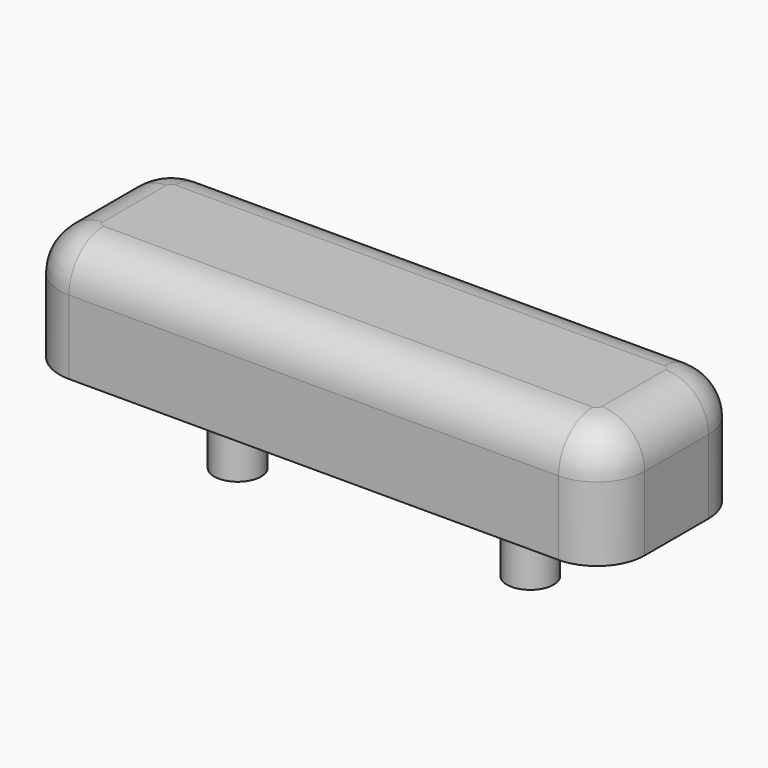
from build123d import *

# Parameters (mm, degrees)
F0_W         = 50
F0_H         = 15
F0_R         = 2
F1_DEPTH     = 10
F2_R         = 3.6792614691
F3_T1_DEPTH  = 20.2290713461
F3_T4_ANGLE  = 90
F3_T6_ANGLE  = 90
F3_T8_ANGLE  = 90
F3_T10_ANGLE = 90
F4_D         = 4.5
F4_DEPTH     = 0.5
F4_TIP       = 1.3519363928
F5_DEPTH     = 7


# Not quite as in the source:
# - a fillet or chamfer that OpenCascade refuses, or shapes differently, is made with other operations: its cross-section is extruded or revolved along the edge and cut away or added


with BuildPart() as f1:
    # F0 (on Top) → F1 (new body)
    with BuildSketch(Plane.XY):
        Rectangle(F0_W, F0_H)
        with Locations((-12.5, 0)):
            Circle(F0_R, mode=Mode.SUBTRACT)
        with Locations((12.5, 0)):
            Circle(F0_R, mode=Mode.SUBTRACT)
        with Locations((12.5, 0)):
            Circle(F0_R)
        with Locations((-12.5, 0)):
            Circle(F0_R)
    extrude(amount=F1_DEPTH)

    # F2
    f2_edges = [f1.edges().sort_by_distance(p)[0] for p in [
        (0, -7.5, 10),
        (-25, 0, 10),
        (25, 0, 10),
        (0, 7.5, 10),
    ]]
    fillet(f2_edges, radius=F2_R)

    # F3: fillet of radius 4.0916285384 on 4 edges, made by hand

    # F3_s2 → F3_t1 (cut)
    with BuildSketch(Plane.XY.offset(-10.2290713461)):
        with BuildLine():
            ThreePointArc((-20.9083714616, 7.5), (-23.8015897472, 6.3015897472), (-25, 3.4083714616))
            Line((-25, 3.4083714616), (-25, 7.5))
            Line((-25, 7.5), (-20.9083714616, 7.5))
        make_face()
        with BuildLine():
            ThreePointArc((-20.9083714616, -7.5), (-23.8015897472, -6.3015897472), (-25, -3.4083714616))
            Line((-25, -3.4083714616), (-25, -7.5))
            Line((-25, -7.5), (-20.9083714616, -7.5))
        make_face()
        with BuildLine():
            ThreePointArc((25, 3.4083714616), (23.8015897472, 6.3015897472), (20.9083714616, 7.5))
            Line((20.9083714616, 7.5), (25, 7.5))
            Line((25, 7.5), (25, 3.4083714616))
        make_face()
        with BuildLine():
            ThreePointArc((25, -3.4083714616), (23.8015897472, -6.3015897472), (20.9083714616, -7.5))
            Line((20.9083714616, -7.5), (25, -7.5))
            Line((25, -7.5), (25, -3.4083714616))
        make_face()
    extrude(amount=F3_T1_DEPTH, mode=Mode.SUBTRACT)

    # F3_s3 → F3_t4 (revolve, cut)
    with BuildSketch(Plane.YZ.offset(20.9083714616)):
        with BuildLine():
            ThreePointArc((-3.8207385309, 10), (-6.4223692655, 8.9223692655), (-7.5, 6.3207385309))
            Line((-7.5, 6.3207385309), (-7.5, 10))
            Line((-7.5, 10), (-3.8207385309, 10))
        make_face()
    revolve(axis=Axis((20.9083714616, -3.4083714616, 10), (0, 0, 1)), revolution_arc=F3_T4_ANGLE, mode=Mode.SUBTRACT)

    # F3_s5 → F3_t6 (revolve, cut)
    with BuildSketch(Plane.XZ.offset(-3.4083714616)):
        with BuildLine():
            ThreePointArc((21.3207385309, 10), (23.9223692655, 8.9223692655), (25, 6.3207385309))
            Line((25, 6.3207385309), (25, 10))
            Line((25, 10), (21.3207385309, 10))
        make_face()
    revolve(axis=Axis((20.9083714616, 3.4083714616, 10), (0, 0, 1)), revolution_arc=F3_T6_ANGLE, mode=Mode.SUBTRACT)

    # F3_s7 → F3_t8 (revolve, cut)
    with BuildSketch(Plane.XZ.offset(3.4083714616)):
        with BuildLine():
            ThreePointArc((-21.3207385309, 10), (-23.9223692655, 8.9223692655), (-25, 6.3207385309))
            Line((-25, 6.3207385309), (-25, 10))
            Line((-25, 10), (-21.3207385309, 10))
        make_face()
    revolve(axis=Axis((-20.9083714616, -3.4083714616, 10), (0, 0, 1)), revolution_arc=F3_T8_ANGLE, mode=Mode.SUBTRACT)

    # F3_s9 → F3_t10 (revolve, cut)
    with BuildSketch(Plane.YZ.offset(-20.9083714616)):
        with BuildLine():
            ThreePointArc((3.8207385309, 10), (6.4223692655, 8.9223692655), (7.5, 6.3207385309))
            Line((7.5, 6.3207385309), (7.5, 10))
            Line((7.5, 10), (3.8207385309, 10))
        make_face()
    revolve(axis=Axis((-20.9083714616, 3.4083714616, 10), (0, 0, 1)), revolution_arc=F3_T10_ANGLE, mode=Mode.SUBTRACT)

    # F4
    with Locations(Plane(origin=(0, 0, 0), x_dir=(1, 0, 0), z_dir=(0, 0, -1))):
        with Locations((0, 0)):
            Hole(F4_D / 2, depth=F4_DEPTH)
            with Locations((0, 0, -(F4_DEPTH + F4_TIP / 2))):  # 118° drill point
                Cone(0, F4_D / 2, F4_TIP, mode=Mode.SUBTRACT)

    # F0 (on Top) → F5 (join)
    with BuildSketch(Plane.XY):
        with Locations((12.5, 0)):
            Circle(F0_R)
        with Locations((-12.5, 0)):
            Circle(F0_R)
    extrude(amount=-F5_DEPTH)


solid = f1.part
